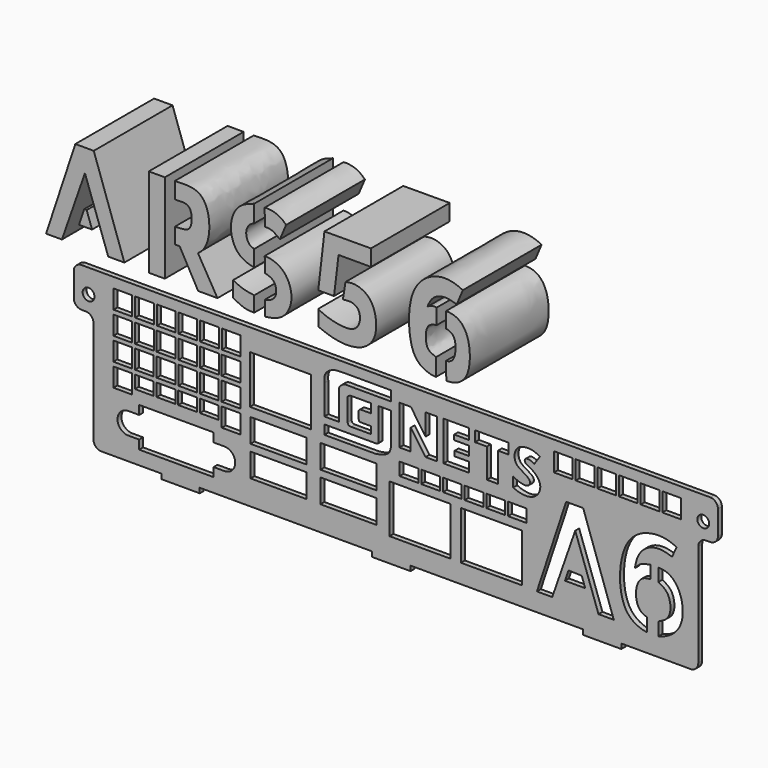
from build123d import *

# Parameters (mm, degrees)
F0_W     = 4.8303119838
F0_H     = 4.8303129151
F0_H_2   = 3.302
F0_W_2   = 14.478
F0_H_3   = 6.096
F0_W_3   = 15.748
F0_H_4   = 12.446
F0_R     = 1.524
F1_DEPTH = 1.27
F3_DEPTH = 25.4
F2_W     = 4.1400529444
F2_H     = 23.0146273971


# Not quite as in the source:
# - a feature names something its author has since deleted; it is built from what else it names


with BuildPart() as f1:
    # F0 (on Front) → F1 (new body)
    with BuildSketch(Plane.XZ):
        with BuildLine():
            Line((-78.5494650882, -42.7973051389), (-78.6328772508, -38.6520951476))
            Line((-78.6328772508, -38.6520951476), (-78.6328772508, -42.2257361916))
            ThreePointArc((-78.6328772508, -42.2257361916), (-78.6119143493, -42.5145478302), (-78.5494650882, -42.7973051389))
        make_face()
        with BuildLine():
            Line((77.3231227492, -3.5857361916), (-78.6328772508, -3.5857361916))
            Line((-78.6328772508, -3.5857361916), (-81.7128772508, -3.5857361916))
            ThreePointArc((-81.7128772508, -3.5857361916), (-83.1270908132, -4.1715226292), (-83.7128772508, -5.5857361916))
            Line((-83.7128772508, -5.5857361916), (-83.7128772508, -11.7457361916))
            ThreePointArc((-83.7128772508, -11.7457361916), (-83.1270908132, -13.1599497539), (-81.7128772508, -13.7457361916))
            Line((-81.7128772508, -13.7457361916), (-80.6328772508, -13.7457361916))
            ThreePointArc((-80.6328772508, -13.7457361916), (-79.2186636884, -14.3315226292), (-78.6328772508, -15.7457361916))
            Line((-78.6328772508, -15.7457361916), (-78.6328772508, -38.6520951476))
            Line((-78.6328772508, -38.6520951476), (-78.5494650882, -42.7973051389))
            ThreePointArc((-78.5494650882, -42.7973051389), (-77.8280471352, -43.8293474123), (-76.6328772508, -44.2257361916))
            Line((-76.6328772508, -44.2257361916), (-61.1388772508, -44.2257361916))
            Line((-61.1388772508, -44.2257361916), (-61.1388772508, -45.4957361916))
            Line((-61.1388772508, -45.4957361916), (-51.2328772508, -45.4957361916))
            Line((-51.2328772508, -45.4957361916), (-51.2328772508, -44.2257361916))
            Line((-51.2328772508, -44.2257361916), (-6.7828772508, -44.2257361916))
            Line((-6.7828772508, -44.2257361916), (-6.7828772508, -45.4957361916))
            Line((-6.7828772508, -45.4957361916), (3.1231227492, -45.4957361916))
            Line((3.1231227492, -45.4957361916), (3.1231227492, -44.2257361916))
            Line((3.1231227492, -44.2257361916), (47.5731227492, -44.2257361916))
            Line((47.5731227492, -44.2257361916), (47.5731227492, -45.4957361916))
            Line((47.5731227492, -45.4957361916), (57.4791227492, -45.4957361916))
            Line((57.4791227492, -45.4957361916), (57.4791227492, -44.2257361916))
            Line((57.4791227492, -44.2257361916), (75.3231227492, -44.2257361916))
            ThreePointArc((75.3231227492, -44.2257361916), (76.7373363116, -43.6399497539), (77.3231227492, -42.2257361916))
            Line((77.3231227492, -42.2257361916), (77.3231227492, -15.7457361916))
            ThreePointArc((77.3231227492, -15.7457361916), (77.9089091868, -14.3315226292), (79.3231227492, -13.7457361916))
            Line((79.3231227492, -13.7457361916), (80.4031227492, -13.7457361916))
            ThreePointArc((80.4031227492, -13.7457361916), (81.8173363116, -13.1599497539), (82.4031227492, -11.7457361916))
            Line((82.4031227492, -11.7457361916), (82.4031227492, -7.6598536155))
            Line((82.4031227492, -7.6598536155), (82.4031227492, -5.5857361916))
            ThreePointArc((82.4031227492, -5.5857361916), (81.8173363116, -4.1715226292), (80.4031227492, -3.5857361916))
            Line((80.4031227492, -3.5857361916), (77.3231227492, -3.5857361916))
        make_face()
        with BuildLine():
            Line((-66.8496239283, -32.7857362416), (-66.8496239283, -30.4997362416))
            Line((-66.8496239283, -30.4997362416), (-47.6726239283, -30.4997362416))
            Line((-47.6726239283, -30.4997362416), (-47.6726239283, -32.7857362416))
            Line((-47.6726239283, -32.7857362416), (-44.8786239283, -32.7857362416))
            ThreePointArc((-44.8786239283, -32.7857362416), (-42.0846239283, -35.5797362416), (-44.8786239283, -38.3737362416))
            Line((-44.8786239283, -38.3737362416), (-47.6726239283, -38.3737362416))
            Line((-47.6726239283, -38.3737362416), (-47.6726239283, -40.6597362416))
            Line((-47.6726239283, -40.6597362416), (-66.8496239283, -40.6597362416))
            Line((-66.8496239283, -40.6597362416), (-66.8496239283, -38.3737362416))
            Line((-66.8496239283, -38.3737362416), (-69.6436239283, -38.3737362416))
            ThreePointArc((-69.6436239283, -38.3737362416), (-72.4376239283, -35.5797362416), (-69.6436239283, -32.7857362416))
            Line((-69.6436239283, -32.7857362416), (-66.8496239283, -32.7857362416))
        make_face(mode=Mode.SUBTRACT)
        with Locations((-71.0845588452, -26.345167762)):
            Rectangle(F0_W, F0_H, mode=Mode.SUBTRACT)
        with Locations((-65.5439929769, -25.6112124523)):
            Rectangle(F0_W, F0_H_2, mode=Mode.SUBTRACT)
        with Locations((-59.9559929769, -25.6112124523)):
            Rectangle(F0_W, F0_H_2, mode=Mode.SUBTRACT)
        with Locations((-54.3679929769, -25.6112124523)):
            Rectangle(F0_W, F0_H_2, mode=Mode.SUBTRACT)
        with Locations((-43.1443509402, -26.3363585101)):
            Rectangle(F0_W, F0_H, mode=Mode.SUBTRACT)
        with Locations((-48.7799929769, -25.6112124523)):
            Rectangle(F0_W, F0_H_2, mode=Mode.SUBTRACT)
        with Locations((-30.8923767439, -34.8023361916)):
            Rectangle(F0_W_2, F0_H_3, mode=Mode.SUBTRACT)
        with Locations((-12.8583767439, -34.8023361916)):
            Rectangle(F0_W_2, F0_H_3, mode=Mode.SUBTRACT)
        with Locations((-30.9134061676, -26.9537361916)):
            Rectangle(F0_W_2, F0_H_3, mode=Mode.SUBTRACT)
        with Locations((-12.8794061676, -26.9537361916)):
            Rectangle(F0_W_2, F0_H_3, mode=Mode.SUBTRACT)
        with Locations((5.5853361653, -33.0859759047)):
            Rectangle(F0_W_3, F0_H_4, mode=Mode.SUBTRACT)
        with Locations((23.9746443206, -33.1303918861)):
            Rectangle(F0_W_3, F0_H_4, mode=Mode.SUBTRACT)
        Polygon((42.9549021294, -34.7071158803), (43.8331411799, -32.0723987288), (47.2651366566, -32.14827681), (48.1511475166, -34.7071158803), align=None, mode=Mode.SUBTRACT)
        with BuildLine():
            Line((67.0504957212, -27.1689015544), (67.0504957212, -23.8755083746))
            add(Edge.make_bspline(
                [(67.0504957212, -23.8755083746), (68.8801608754, -23.8755083746), (71.7782886169, -25.346447245), (73.7971156732, -30.8843605661), (72.7390189302, -36.9577562984), (68.8706348161, -39.0836969495), (67.0504957212, -39.4867127351)],
                knots=[0, 0, 0, 0, 0.2321387928, 0.4843476193, 0.7416743379, 1, 1, 1, 1], degree=3))
            Line((67.0504957212, -39.4867127351), (67.0504957212, -36.0976587153))
            add(Edge.make_bspline(
                [(67.0504957212, -27.1689015544), (68.0063732883, -27.6892859229), (70.1068037799, -28.8327704366), (70.5014219766, -34.4849615135), (68.1399999091, -35.5885083524), (67.0504957212, -36.0976587153)],
                knots=[0, 0, 0, 0, 0.3102656516, 0.681772915, 1, 1, 1, 1], degree=3))
        make_face(mode=Mode.SUBTRACT)
        Polygon((39.6588149704, -39.4867127351), (35.7068822363, -39.4867127351), (43.2481538909, -16.6814267326), (47.635636736, -16.6814267326), (55.5320813772, -39.4867127351), (51.5936401786, -39.4867127351), (45.5896174183, -22.4849618143), align=None, mode=Mode.SUBTRACT)
        with BuildLine():
            add(Edge.make_bspline(
                [(71.7401202823, -17.7273699299), (69.6162202447, -16.6814267326), (65.5033349496, -16.011376397), (56.7668670803, -19.8199474552), (56.3250657345, -37.8039324123), (63.6486503932, -39.5380594106), (64.0698431812, -39.49887601), (64.1104905305, -39.4867127351)],
                knots=[0, 0, 0, 0, 0.2054191626, 0.4393093006, 0.7619425743, 0.9558214245, 1, 1, 1, 1], degree=3))
            Line((71.7401202823, -17.7273699299), (70.5634519233, -20.2893651194))
            add(Edge.make_bspline(
                [(70.5634519233, -20.2893651194), (69.2033885172, -19.8043901938), (66.5575951938, -19.1889542175), (62.4234432355, -20.9757381456), (61.233105858, -24.0680686804), (60.9760150088, -25.9979180163)],
                knots=[0, 0, 0, 0, 0.3223796569, 0.6400919097, 1, 1, 1, 1], degree=3))
            add(Edge.make_bspline(
                [(65.0012731327, -23.8755083746), (64.1831867378, -24.0293929875), (62.2850572897, -24.4427552333), (61.7592763525, -25.1434468125), (60.9760150088, -25.9979180163)],
                knots=[0, 0, 0, 0, 0.5175114754, 1, 1, 1, 1], degree=3))
            Line((65.0012731327, -23.8755083746), (65.0012731327, -27.1689015544))
            add(Edge.make_bspline(
                [(65.0012731327, -27.1689015544), (64.1569426892, -27.267745801), (62.2934606831, -27.4859002884), (60.8259642773, -31.1644342823), (61.8070124123, -35.3079162938), (63.4207458547, -35.8611812657), (64.1104905305, -36.0976587153)],
                knots=[0, 0, 0, 0, 0.2264825943, 0.4998590805, 0.7862289227, 1, 1, 1, 1], degree=3))
            Line((64.1104905305, -36.0976587153), (64.1104905305, -39.4867127351))
        make_face(mode=Mode.SUBTRACT)
        with Locations((-71.1063830419, -20.4488243877)):
            Rectangle(F0_W, F0_H, mode=Mode.SUBTRACT)
        with Locations((-65.5183830419, -20.4488243877)):
            Rectangle(F0_W, F0_H, mode=Mode.SUBTRACT)
        with Locations((-59.9303830419, -20.4488243877)):
            Rectangle(F0_W, F0_H, mode=Mode.SUBTRACT)
        with Locations((-54.3423830419, -20.4488243877)):
            Rectangle(F0_W, F0_H, mode=Mode.SUBTRACT)
        with Locations((-48.7543830419, -20.4488243877)):
            Rectangle(F0_W, F0_H, mode=Mode.SUBTRACT)
        with Locations((-43.1663830419, -20.4488243877)):
            Rectangle(F0_W, F0_H, mode=Mode.SUBTRACT)
        with Locations((-71.0890587338, -14.5649888681)):
            Rectangle(F0_W, F0_H, mode=Mode.SUBTRACT)
        with Locations((-65.5010587338, -14.5649888681)):
            Rectangle(F0_W, F0_H, mode=Mode.SUBTRACT)
        with Locations((-59.9130587338, -14.5649888681)):
            Rectangle(F0_W, F0_H, mode=Mode.SUBTRACT)
        with Locations((-54.3250587338, -14.5649888681)):
            Rectangle(F0_W, F0_H, mode=Mode.SUBTRACT)
        with Locations((-48.7370587338, -14.5649888681)):
            Rectangle(F0_W, F0_H, mode=Mode.SUBTRACT)
        with Locations((-43.1490587338, -14.5649888681)):
            Rectangle(F0_W, F0_H, mode=Mode.SUBTRACT)
        with Locations((-30.4301999227, -15.4347545546)):
            Rectangle(F0_W_3, F0_H_4, mode=Mode.SUBTRACT)
        with BuildLine():
            Line((-5.1270304248, -18.8832334552), (-5.1270304248, -12.9603850433))
            Line((-5.1270304248, -12.9603850433), (-5.1270304248, -10.6733843854))
            Line((-5.1270304248, -10.6733843854), (-1.9192821985, -10.6733843854))
            Line((-1.9192821985, -10.6733843854), (-1.9192821985, -18.9073926008))
            add(Edge.make_bspline(
                [(-5.9016659563, -21.7701459474), (-5.4522837178, -21.7077571885), (-4.4595879995, -21.5699389826), (-2.2656727008, -20.7247817822), (-2.0303550209, -19.4901526491), (-1.9192821985, -18.9073926008)],
                knots=[0, 0, 0, 0, 0.3039634344, 0.6714622296, 1, 1, 1, 1], degree=3))
            Line((-5.9016659563, -21.7701459474), (-19.1066188405, -21.7701459474))
            Line((-19.1066188405, -21.7701459474), (-19.1066188405, -19.382035563))
            Line((-19.1066188405, -19.382035563), (-5.6258325326, -19.382035563))
            ThreePointArc((-5.6258325326, -19.382035563), (-5.2731261797, -19.2359398081), (-5.1270304248, -18.8832334552))
        make_face(mode=Mode.SUBTRACT)
        with BuildLine():
            Line((-7.0446659563, -15.8832775314), (-7.0446659563, -17.7005712812))
            Line((-7.0446659563, -17.7005712812), (-12.1266078204, -17.7005712812))
            add(Edge.make_bspline(
                [(-13.0755543416, -16.9791746885), (-13.0708856821, -17.2279909249), (-12.8661300603, -17.6394300283), (-12.4417270045, -17.7120329269), (-12.1266078204, -17.7005712812)],
                knots=[0, 0, 0, 0, 0.4829521491, 1, 1, 1, 1], degree=3))
            Line((-13.0755543416, -16.9791746885), (-13.0755543416, -11.1135014656))
            ThreePointArc((-13.0755543416, -11.1135014656), (-12.6428574052, -10.7886438717), (-12.1142040727, -10.6733843854))
            Line((-12.1142040727, -10.6733843854), (-7.0634005216, -10.6733843854))
            Line((-7.0634005216, -10.6733843854), (-7.0446659563, -12.9759874148))
            Line((-7.0446659563, -12.9759874148), (-9.6341120653, -12.9970558085))
            ThreePointArc((-9.6341120653, -12.9970558085), (-9.9977287409, -13.1068010116), (-10.244644247, -13.3954077149))
            Line((-10.244644247, -13.3954077149), (-10.244644247, -15.3690706939))
            add(Edge.make_bspline(
                [(-10.244644247, -15.3690706939), (-10.2210138111, -15.547179273), (-10.172850174, -15.8949875976), (-9.8142910472, -15.8970843281), (-9.6341120653, -15.8832775314)],
                knots=[0, 0, 0, 0, 0.4989424998, 1, 1, 1, 1], degree=3))
            Line((-9.6341120653, -15.8832775314), (-7.0446659563, -15.8832775314))
        make_face(mode=Mode.SUBTRACT)
        with Locations((-79.9028772508, -9.6817361916)):
            Circle(F0_R, mode=Mode.SUBTRACT)
        with Locations((-71.0634487988, -8.617357261)):
            Rectangle(F0_W, F0_H, mode=Mode.SUBTRACT)
        with Locations((-65.4754487988, -8.617357261)):
            Rectangle(F0_W, F0_H, mode=Mode.SUBTRACT)
        with Locations((-59.8874487988, -8.617357261)):
            Rectangle(F0_W, F0_H, mode=Mode.SUBTRACT)
        with Locations((-54.2994487988, -8.617357261)):
            Rectangle(F0_W, F0_H, mode=Mode.SUBTRACT)
        with Locations((-48.7114487988, -8.617357261)):
            Rectangle(F0_W, F0_H, mode=Mode.SUBTRACT)
        with Locations((-43.1234487988, -8.617357261)):
            Rectangle(F0_W, F0_H, mode=Mode.SUBTRACT)
        with BuildLine():
            Line((-19.1066188405, -17.5989712812), (-19.1066188405, -9.9789712812))
            add(Edge.make_bspline(
                [(-19.1066188405, -9.9789712812), (-19.1499280424, -9.008612815), (-19.1529968051, -7.709668362), (-17.0271997948, -6.1086794595), (-15.4760578426, -6.0952657679), (-14.6192821985, -6.0616467731)],
                knots=[0, 0, 0, 0, 0.327543449, 0.6579258999, 1, 1, 1, 1], degree=3))
            Line((-14.6192821985, -6.0616467731), (-1.9192821985, -6.0616467731))
            Line((-1.9192821985, -6.0616467731), (-1.9192821985, -8.6016467731))
            Line((-1.9192821985, -8.6016467731), (-11.8055543416, -8.6016467731))
            add(Edge.make_bspline(
                [(-11.8055543416, -8.6016467731), (-12.5837568893, -8.6390232057), (-14.0889139528, -8.3062188136), (-15.2954617753, -9.6379536679), (-15.2239041107, -9.6409651333), (-15.2966188405, -9.9789712812)],
                knots=[0, 0, 0, 0, 0.453396986, 0.7992270184, 1, 1, 1, 1], degree=3))
            Line((-15.2966188405, -9.9789712812), (-15.2966188405, -17.5989712812))
            Line((-15.2966188405, -17.5989712812), (-19.1066188405, -17.5989712812))
        make_face(mode=Mode.SUBTRACT)
        with Locations((2.7129778897, -23.1719435998)):
            Rectangle(F0_W, F0_H_2, mode=Mode.SUBTRACT)
        with Locations((8.3009778897, -23.1719435998)):
            Rectangle(F0_W, F0_H_2, mode=Mode.SUBTRACT)
        with Locations((13.8889778897, -23.1719435998)):
            Rectangle(F0_W, F0_H_2, mode=Mode.SUBTRACT)
        with Locations((19.4769778897, -23.1719435998)):
            Rectangle(F0_W, F0_H_2, mode=Mode.SUBTRACT)
        with Locations((25.0649778897, -23.1719435998)):
            Rectangle(F0_W, F0_H_2, mode=Mode.SUBTRACT)
        with Locations((30.6529778897, -23.1719435998)):
            Rectangle(F0_W, F0_H_2, mode=Mode.SUBTRACT)
        Polygon((3.170271854, -18.3332680965), (0.2606075123, -18.3332680965), (0.2606075123, -8.1595447894), (3.2112535654, -8.1595447894), (6.9815264129, -13.7043710906), (6.9815264129, -8.1595447894), (9.9321761828, -8.1595447894), (9.9321761828, -18.3332680965), (6.9815264129, -18.3332680965), (3.170271854, -12.8847442961), align=None, mode=Mode.SUBTRACT)
        Polygon((11.620653416, -18.2572412543), (11.620653416, -8.0835179472), (18.2351243097, -8.0835179472), (18.2351243097, -10.8147732263), (14.3670116218, -10.8147732263), (14.3670116218, -12.0912507665), (18.2351243097, -12.0912507665), (18.2351243097, -14.4507985397), (14.4830564706, -14.4507985397), (14.4830564706, -15.7272756153), (18.2351243097, -15.7272756153), (18.2351243097, -18.2572412543), align=None, mode=Mode.SUBTRACT)
        Polygon((19.7626439966, -10.7978000949), (19.7626439966, -8.0862555751), (28.4106183691, -8.0862555751), (28.4106183691, -10.7978000949), (25.6506266173, -10.7978000949), (25.6506266173, -18.3417773486), (22.7986339247, -18.3417773486), (22.7986339247, -10.7978000949), align=None, mode=Mode.SUBTRACT)
        with BuildLine():
            add(Edge.make_bspline(
                [(35.0518489116, -10.7536256639), (33.8523346458, -10.0489755714), (32.4962515301, -10.0823113646), (32.5587022819, -11.4059684081), (34.1943205562, -12.0841749793), (35.9122419379, -13.2939228916), (36.9051523771, -15.4328377818), (35.9319633391, -17.8974196347), (33.5159920428, -18.9165376462), (31.155264137, -18.4920988903), (30.4147554067, -18.280419797), (29.5984597736, -17.8923618945)],
                knots=[0, 0, 0, 0, 0.1228250476, 0.1926608238, 0.2950367563, 0.4114467783, 0.5286176392, 0.6509011519, 0.7761394901, 0.8931483505, 1, 1, 1, 1], degree=3))
            Line((29.5984597736, -17.8923618945), (29.5984597736, -15.3702761012))
            add(Edge.make_bspline(
                [(36.4710051591, -8.6470655424), (35.1109534025, -7.8310337567), (33.3976823718, -7.5326005666), (30.8994687371, -8.0541921441), (29.8175765565, -9.767137269), (29.9981021978, -12.2398137788), (31.9068575422, -13.4588557868), (34.3296412665, -14.7980446241), (33.5585513611, -16.6654827192), (30.988053932, -16.1526203591), (30.3644832615, -15.752474662), (29.5984597736, -15.3702761012)],
                knots=[0, 0, 0, 0, 0.1399276033, 0.2530861684, 0.356009097, 0.4680148146, 0.5822310701, 0.7012342568, 0.786771174, 0.8981655597, 1, 1, 1, 1], degree=3))
            Line((36.4710051591, -8.6470655424), (35.0518489116, -10.7536256639))
        make_face(mode=Mode.SUBTRACT)
        with Locations((78.6059464398, -9.6664536155)):
            Circle(F0_R, mode=Mode.SUBTRACT)
        with Locations((42.5270227482, -8.6387255516)):
            Rectangle(F0_W, F0_H, mode=Mode.SUBTRACT)
        with Locations((48.1150227482, -8.6387255516)):
            Rectangle(F0_W, F0_H, mode=Mode.SUBTRACT)
        with Locations((53.7030227482, -8.6387255516)):
            Rectangle(F0_W, F0_H, mode=Mode.SUBTRACT)
        with Locations((59.2910227482, -8.6387255516)):
            Rectangle(F0_W, F0_H, mode=Mode.SUBTRACT)
        with Locations((64.8790227482, -8.6387255516)):
            Rectangle(F0_W, F0_H, mode=Mode.SUBTRACT)
        with Locations((70.4670227482, -8.6387255516)):
            Rectangle(F0_W, F0_H, mode=Mode.SUBTRACT)
    extrude(amount=F1_DEPTH)


with BuildPart() as f3:
    # F2 (on Front) → F3 (new body)
    with BuildSketch(Plane.XZ):
        Polygon((-64.0139225292, 39.4597202282), (-71.5551941838, 16.6544342256), (-67.465524534, 16.6544342256), (-61.5347220862, 33.6561851464), (-55.5306993259, 16.6544342256), (-51.3654696743, 16.6544342256), (-59.2619143155, 39.4597202282), align=None)
    extrude(amount=F3_DEPTH)


with BuildPart() as f3b:
    # F2 (on Front) → F3, piece 2 (new body)
    with BuildSketch(Plane.XZ):
        Polygon((-61.0837050083, 25.4156338885), (-61.7153908129, 25.4295998471), (-63.0472470685, 21.4340310805), (-59.7050550693, 21.4340310805), align=None)
    extrude(amount=F3_DEPTH)


with BuildPart() as f3c:
    # F2 (on Front) → F3, piece 3 (new body)
    with BuildSketch(Plane.XZ):
        with BuildLine():
            Line((-11.2564321607, 34.9926277995), (-9.6621618825, 38.7644037135))
            add(Edge.make_bspline(
                [(-9.6621618825, 38.7644037135), (-10.4734370798, 39.5805638424), (-11.7170521192, 40.530501587), (-14.0666486695, 41.0244613886), (-15.1703245938, 40.9082882106)],
                knots=[0, 0, 0, 0, 0.4786637371, 1, 1, 1, 1], degree=3))
            Line((-15.1703245938, 40.9082882106), (-15.1601622587, 36.5804746667))
            add(Edge.make_bspline(
                [(-11.2564321607, 34.9926277995), (-11.9578751075, 35.4958464126), (-13.191923315, 36.5496209128), (-14.5536134169, 36.5454382543), (-15.1601622587, 36.5804746667)],
                knots=[0, 0, 0, 0, 0.5337181975, 1, 1, 1, 1], degree=3))
        make_face()
    extrude(amount=F3_DEPTH)


with BuildPart() as f3d:
    # F2 (on Front) → F3, piece 4 (new body)
    with BuildSketch(Plane.XZ):
        with BuildLine():
            Line((-23.2970804055, 21.8210662729), (-23.3194609492, 17.7398286294))
            add(Edge.make_bspline(
                [(-23.3194609492, 17.7398286294), (-22.286867998, 17.195076324), (-20.3754891592, 16.1867138054), (-18.6710768598, 16.1702742098), (-17.8874470294, 16.1627158523)],
                knots=[0, 0, 0, 0, 0.5402345837, 1, 1, 1, 1], degree=3))
            Line((-17.8874470294, 16.1627158523), (-17.8874470294, 20.1127137989))
            add(Edge.make_bspline(
                [(-23.2970804055, 21.8210662729), (-22.3195415161, 21.2306694641), (-20.4352166764, 20.4870302961), (-19.2064144729, 20.3150523837), (-17.8874470294, 20.1127137989)],
                knots=[0, 0, 0, 0, 0.5115067465, 1, 1, 1, 1], degree=3))
        make_face()
    extrude(amount=F3_DEPTH)


with BuildPart() as f3e:
    # F2 (on Front) → F3, piece 5 (new body)
    with BuildSketch(Plane.XZ):
        Polygon((12.2178126847, 36.3555292649), (12.2178126847, 40.5519942803), (0.2244644378, 40.5041470334), (-1.3663708232, 26.6220439225), (2.6926299951, 26.6220439225), (3.8659489899, 36.3555292649), align=None)
    extrude(amount=F3_DEPTH)


with BuildPart() as f3f:
    # F2 (on Front) → F3, piece 6 (new body)
    with BuildSketch(Plane.XZ):
        with BuildLine():
            Line((5.6606231786, 30.8038893417), (4.9888868816, 26.6220439225))
            add(Edge.make_bspline(
                [(4.9888868816, 26.6220439225), (5.9766980191, 26.6721323843), (7.0076021873, 26.9059624848), (9.3149315177, 25.9319288635), (9.5897650725, 22.7756978079), (8.2021362436, 20.7755805771), (5.5155990376, 20.1467171271), (0.7881518583, 21.0681352435), (-1.3663708232, 22.4147119496)],
                knots=[0, 0, 0, 0, 0.1416298525, 0.279703447, 0.4425002776, 0.5850456501, 0.7386780043, 1, 1, 1, 1], degree=3))
            Line((-1.3663708232, 22.4147119496), (-1.3663708232, 18.3638560636))
            add(Edge.make_bspline(
                [(-1.3663708232, 18.3638560636), (0.2871224522, 17.7112345801), (3.7335525237, 16.4279257338), (9.8894762556, 16.6138193365), (13.742349257, 20.306232142), (13.6662200515, 25.9671411085), (11.7711664945, 29.8683309484), (8.1038213142, 31.2631388213), (6.6179329333, 30.9870969956), (5.6606231786, 30.8038893417)],
                knots=[0, 0, 0, 0, 0.1586880914, 0.3227517855, 0.4706525111, 0.6272466396, 0.7660149784, 0.8926259982, 1, 1, 1, 1], degree=3))
        make_face()
    extrude(amount=F3_DEPTH)


with BuildPart() as f3g:
    # F2 (on Front) → F3, piece 7 (new body)
    with BuildSketch(Plane.XZ):
        with BuildLine():
            Line((34.3235917389, 35.0258871913), (35.9161496405, 38.7787313497))
            add(Edge.make_bspline(
                [(35.9161496405, 38.7787313497), (33.8958085945, 39.7736755259), (29.5242711511, 40.8028067592), (21.2176238724, 35.4790843984), (21.9595402938, 19.947536315), (26.1624250277, 17.3978028793), (27.8969753883, 16.8347131082), (29.0047948793, 16.8347131082)],
                knots=[0, 0, 0, 0, 0.1944143578, 0.4199527234, 0.710678892, 0.8696178858, 1, 1, 1, 1], degree=3))
            Line((29.0047948793, 16.8347131082), (29.0047948793, 21.3335100561))
            add(Edge.make_bspline(
                [(29.1688672023, 28.6361109465), (28.2677115483, 28.5306142747), (26.6004525051, 28.1171904916), (26.1581747346, 24.5804033632), (26.886472622, 22.094797864), (28.0880401023, 21.7264057623), (29.0047948793, 21.3335100561)],
                knots=[0, 0, 0, 0, 0.2417253481, 0.5246388928, 0.7661672097, 1, 1, 1, 1], degree=3))
            Line((29.1688672023, 28.6361109465), (29.1688672023, 32.6320249954))
            add(Edge.make_bspline(
                [(29.1688672023, 32.6320249954), (28.4010468665, 32.7482823102), (27.8219138523, 32.5606329153), (27.4444921211, 32.5290388484), (26.7358664423, 32.0136770606)],
                knots=[0, 0, 0, 0, 0.5021789807, 1, 1, 1, 1], degree=3))
            add(Edge.make_bspline(
                [(34.3235917389, 35.0258871913), (32.7513058437, 35.5865369607), (30.6828202045, 35.8545388693), (28.0864476181, 34.7072542356), (27.3213591427, 33.3310328424), (26.7358664423, 32.0136770606)],
                knots=[0, 0, 0, 0, 0.3726833508, 0.6655725511, 1, 1, 1, 1], degree=3))
        make_face()
    extrude(amount=F3_DEPTH)


with BuildPart() as f3h:
    # F2 (on Front) → F3, piece 8 (new body)
    with BuildSketch(Plane.XZ):
        with BuildLine():
            add(Edge.make_bspline(
                [(31.5851159394, 32.6320249954), (33.5140341693, 32.6136808119), (36.3180005208, 31.270203094), (38.1083133591, 25.9051825837), (37.4187764277, 18.2227574245), (33.5422280832, 16.7540611133), (31.6503159702, 16.8347131082)],
                knots=[0, 0, 0, 0, 0.2284844006, 0.4748089213, 0.7574109715, 1, 1, 1, 1], degree=3))
            Line((31.5851159394, 32.6320249954), (31.5851159394, 28.6361109465))
            add(Edge.make_bspline(
                [(31.5851159394, 28.6361109465), (32.5541943312, 28.427535668), (34.2542084772, 27.6303527644), (34.0661088312, 22.2637824473), (32.6273813844, 21.4016269892), (31.5851159394, 21.3335100561)],
                knots=[0, 0, 0, 0, 0.30144459, 0.7061866474, 1, 1, 1, 1], degree=3))
            Line((31.5851159394, 21.3335100561), (31.6503159702, 16.8347131082))
        make_face()
    extrude(amount=F3_DEPTH)


with BuildPart() as f3i:
    # F2 (on Front) → F3, piece 9 (new body)
    with BuildSketch(Plane.XZ):
        with Locations((-43.0009756237, 27.8986177475)):
            Rectangle(F2_W, F2_H)
    extrude(amount=F3_DEPTH)


with BuildPart() as f3j:
    # F2 (on Front) → F3, piece 10 (new body)
    with BuildSketch(Plane.XZ):
        with BuildLine():
            add(Edge.make_bspline(
                [(-38.3656062186, 39.4059314461), (-35.762307444, 39.5322641624), (-30.3901499196, 39.8502460315), (-28.7284231973, 30.2878483626), (-30.6870523605, 26.0850388184), (-32.3951467872, 24.9980694683)],
                knots=[0, 0, 0, 0, 0.3303847916, 0.6864595585, 1, 1, 1, 1], degree=3))
            Line((-38.3656062186, 39.4059314461), (-38.3656062186, 35.2235852809))
            add(Edge.make_bspline(
                [(-38.3656062186, 35.2235852809), (-36.3450997683, 35.3108772409), (-33.8407416719, 35.476906918), (-33.7989189748, 28.9016071595), (-36.4241147236, 29.1918606777), (-38.3656062186, 29.0300703676)],
                knots=[0, 0, 0, 0, 0.3277673895, 0.6706574409, 1, 1, 1, 1], degree=3))
            Line((-38.3656062186, 29.0300703676), (-38.3656062186, 24.9980694683))
            Line((-38.3656062186, 24.9980694683), (-37.104813735, 24.9980694683))
            Line((-37.104813735, 24.9980694683), (-32.3345122818, 16.391304049))
            Line((-32.3345122818, 16.391304049), (-27.3551475257, 16.391304049))
            Line((-27.3551475257, 16.391304049), (-32.3951467872, 24.9980694683))
        make_face()
    extrude(amount=F3_DEPTH)


with BuildPart() as f3k:
    # F2 (on Front) → F3, piece 11 (new body)
    with BuildSketch(Plane.XZ):
        with BuildLine():
            Line((-15.1122361422, 20.0546253473), (-15.1122361422, 16.1702742098))
            add(Edge.make_bspline(
                [(-15.1122361422, 16.1702742098), (-14.1956398619, 16.2467994422), (-12.0940782104, 16.6558851792), (-9.5232080825, 18.2256798835), (-7.5473870024, 22.6263605962), (-9.7303256889, 28.7997026088), (-13.7126830414, 29.9296174198), (-15.1703245938, 29.9296174198)],
                knots=[0, 0, 0, 0, 0.1687767539, 0.335029246, 0.541383466, 0.7802660456, 1, 1, 1, 1], degree=3))
            Line((-15.1703245938, 29.9296174198), (-15.1354646495, 26.0625526807))
            add(Edge.make_bspline(
                [(-15.1122361422, 20.0546253473), (-14.2205950819, 20.1245550826), (-11.8641652413, 21.0068788642), (-12.2670747452, 25.2542894796), (-14.2052352341, 25.7960972952), (-15.1354646495, 26.0625526807)],
                knots=[0, 0, 0, 0, 0.3294738559, 0.6810532821, 1, 1, 1, 1], degree=3))
        make_face()
    extrude(amount=F3_DEPTH)


with BuildPart() as f3l:
    # F2 (on Front) → F3, piece 12 (new body)
    with BuildSketch(Plane.XZ):
        with BuildLine():
            Line((-17.8874470294, 36.435496062), (-17.8874470294, 40.9082882106))
            add(Edge.make_bspline(
                [(-17.8874470294, 40.9082882106), (-19.808281445, 40.3122008652), (-22.608630234, 39.0173297177), (-24.4125676139, 33.9310404377), (-22.9823437629, 28.6398886865), (-20.4235741101, 26.9492771515), (-17.8874470294, 26.3912007213)],
                knots=[0, 0, 0, 0, 0.2479140315, 0.4928902496, 0.7389061467, 1, 1, 1, 1], degree=3))
            Line((-17.8874470294, 26.3912007213), (-17.8874470294, 30.63955158))
            add(Edge.make_bspline(
                [(-17.8874470294, 36.435496062), (-18.6020619434, 36.1808253343), (-19.4699357158, 35.5432827152), (-20.2429576569, 33.5693929318), (-19.3253275458, 31.098992054), (-18.4112842134, 30.8305898406), (-17.8874470294, 30.63955158)],
                knots=[0, 0, 0, 0, 0.2450261611, 0.500486193, 0.7804770383, 1, 1, 1, 1], degree=3))
        make_face()
    extrude(amount=F3_DEPTH)


solid = Compound([f1.part, f3.part, f3b.part, f3c.part, f3d.part, f3e.part, f3f.part, f3g.part, f3h.part, f3i.part, f3j.part, f3k.part, f3l.part])
